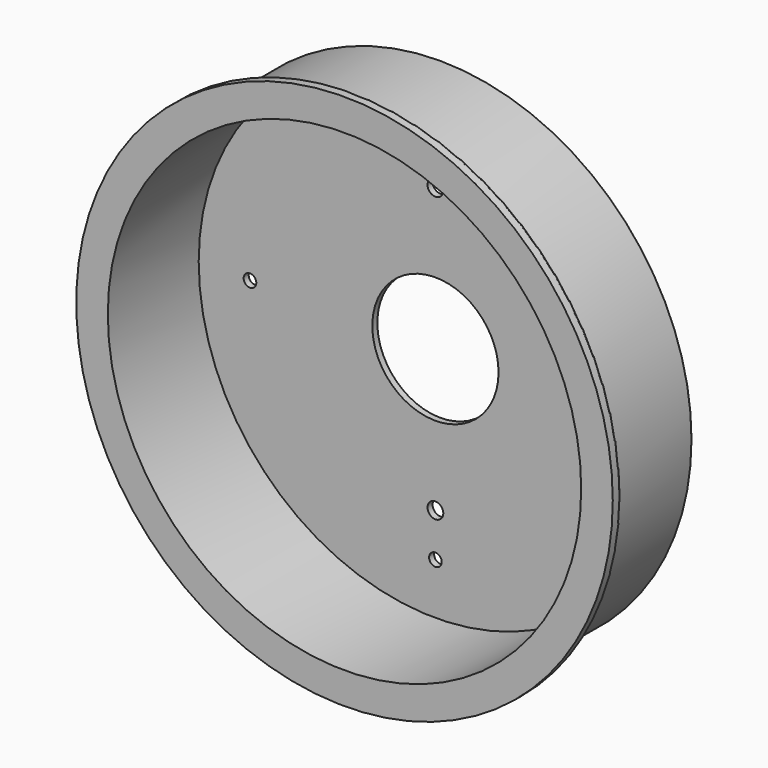
from build123d import *

# Parameters (mm, degrees)
F0_R      = 79.8
F0_R_2    = 20
F1_DEPTH  = 5
F2_R      = 79.8
F2_R_2    = 75
F3_DEPTH  = 30
F4_R      = 85
F4_R_2    = 75
F5_DEPTH  = 3
F7_D      = 5
F7_DEPTH  = 25
F7_TIP    = 1.5021515476
F8_R      = 0.5
F9_DEPTH  = 3
F11_D     = 4
F11_DEPTH = 25
F11_TIP   = 1.2017212381


with BuildPart() as f1:
    # F0 (on Front) → F1 (new body)
    with BuildSketch(Plane.XZ):
        Circle(F0_R)
        Circle(F0_R_2, mode=Mode.SUBTRACT)
    extrude(amount=F1_DEPTH)

    # F2 (on face) → F3 (join)
    with BuildSketch(Plane.XZ.offset(5)):
        Circle(F2_R)
        Circle(F2_R_2, mode=Mode.SUBTRACT)
    extrude(amount=F3_DEPTH)

    # F4 (on face) → F5 (join)
    with BuildSketch(Plane.XZ.offset(35)):
        Circle(F4_R)
        Circle(F4_R_2, mode=Mode.SUBTRACT)
    extrude(amount=F5_DEPTH)

    # F7
    with Locations(Plane(origin=(0, 0, 0), x_dir=(-1, 0, 0), z_dir=(0, 1, 0))):
        with Locations((0, 45), (0, -45)):
            Hole(F7_D / 2, depth=F7_DEPTH)
            with Locations((0, 0, -(F7_DEPTH + F7_TIP / 2))):  # 118° drill point
                Cone(0, F7_D / 2, F7_TIP, mode=Mode.SUBTRACT)

    # F8
    f8_edges = [f1.edges().sort_by_distance(p)[0] for p in [
        (-79.8, 0, 0),
        (-85, -35, 0),
    ]]
    fillet(f8_edges, radius=F8_R)

    # F9 (cut): a face of the model
    f9_faces = [f1.faces().sort_by_distance(p)[0] for p in [
        (-72.8786796564, -5, 0),
    ]]
    extrude(f9_faces, amount=-F9_DEPTH, mode=Mode.SUBTRACT)

    # F11
    with Locations(Plane(origin=(0, 0, 0), x_dir=(-1, 0, 0), z_dir=(0, 1, 0))):
        with Locations((-58.75, 0), (0, 58.75), (58.75, 0), (0, -58.75)):
            Hole(F11_D / 2, depth=F11_DEPTH)
            with Locations((0, 0, -(F11_DEPTH + F11_TIP / 2))):  # 118° drill point
                Cone(0, F11_D / 2, F11_TIP, mode=Mode.SUBTRACT)


solid = f1.part
